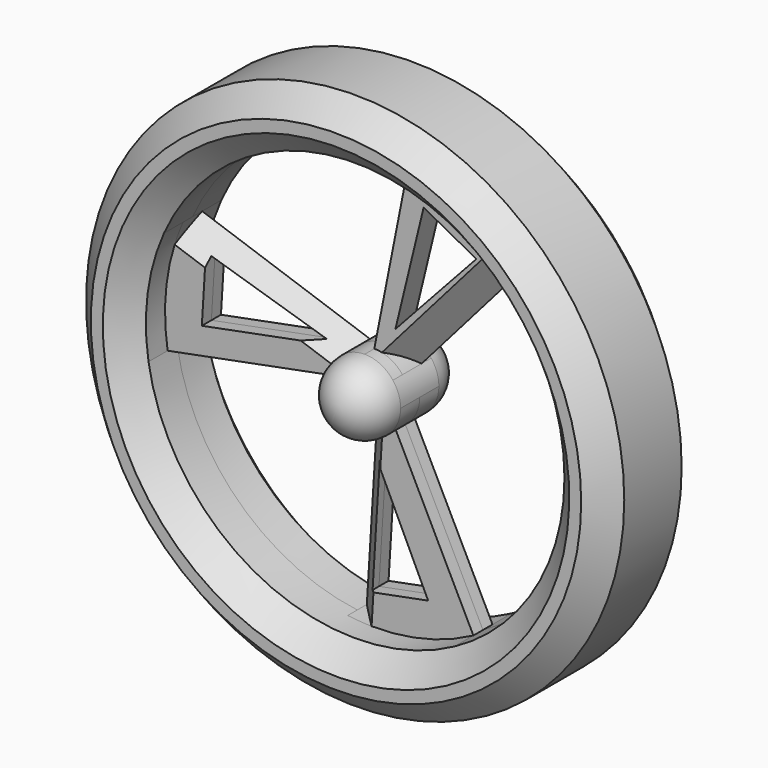
from build123d import *

# Parameters (mm, degrees)
F0_R          = 57.15
F1_DEPTH      = 12.7
F1_DEPTH_BACK = 12.7
F2_DEPTH      = 2.54
F2_DEPTH_BACK = 2.54
F4_T3_DEPTH   = 63.8207499086
F4_S4_R       = 7.62
F4_T5_DEPTH   = 35
F4_S6_R       = 44.45
F4_T7_DEPTH   = 35
F4_T10_DEPTH  = 63.0657347927
F4_S11_R      = 7.62
F4_T12_DEPTH  = 36
F4_S13_R      = 44.45
F4_T14_DEPTH  = 36
F4_T17_DEPTH  = 63.4473233417
F4_S18_R      = 7.62
F4_T19_DEPTH  = 34
F4_S20_R      = 44.45
F4_T21_DEPTH  = 34


# Not quite as in the source:
# - a fillet or chamfer that OpenCascade refuses, or shapes differently, is made with other operations: its cross-section is extruded or revolved along the edge and cut away or added


with BuildPart() as f1:
    # F0 (on Front) → F1 (new body, two sides)
    with BuildSketch(Plane.XZ) as f1_sk:
        Circle(F0_R)
        with BuildLine():
            ThreePointArc((30.2978338322, 32.5245102204), (40.7586875024, 17.7350470278), (44.45, 0))
            ThreePointArc((44.45, 0), (38.1514443262, -22.8094233996), (21.0407853398, -39.1546657793))
            ThreePointArc((21.0407853398, -39.1546657793), (8.0824234514, -43.7090028616), (-5.6476952972, -44.0897498046))
            ThreePointArc((-5.6476952972, -44.0897498046), (-30.9360762044, -31.9180464483), (-43.8918074796, -7.0222315665))
            ThreePointArc((-43.8918074796, -7.0222315665), (-44.0755738858, 5.7572811841), (-40.6153867658, 18.0608100003))
            ThreePointArc((-40.6153867658, 18.0608100003), (-21.1284803601, 39.1074138454), (7.15605679, 43.8701874992))
            ThreePointArc((7.15605679, 43.8701874992), (19.5673089339, 39.9114384743), (30.2978338322, 32.5245102204))
        make_face(mode=Mode.SUBTRACT)
    extrude(amount=F1_DEPTH)
    extrude(f1_sk.sketch, amount=-F1_DEPTH_BACK)



with BuildPart() as f1b:
    # F0 (on Front) → F1, piece 2 (new body, two sides)
    with BuildSketch(Plane.XZ) as f1_2_sk:
        with BuildLine():
            ThreePointArc((7.62, 0), (7.1992672661, 2.4969883522), (5.9835299656, 4.7182379285))
            ThreePointArc((5.9835299656, 4.7182379285), (3.3250133071, 6.8562880998), (0, 7.62))
            ThreePointArc((0, 7.62), (-2.66023415, 7.1405569998), (-4.9857096013, 5.7625601751))
            ThreePointArc((-4.9857096013, 5.7625601751), (-6.930205883, 3.168066669), (-7.62, 0))
            ThreePointArc((-7.62, 0), (-6.4667392377, -4.030593459), (-3.3560410415, -6.8411540348))
            ThreePointArc((-3.3560410415, -6.8411540348), (0.7135883563, -7.5865138013), (4.5728511754, -6.0953615256))
            ThreePointArc((4.5728511754, -6.0953615256), (6.815773102, -3.407291743), (7.62, 0))
        make_face()
    extrude(amount=F1_DEPTH)
    extrude(f1_2_sk.sketch, amount=-F1_DEPTH_BACK)


with BuildPart() as f1_1:
    add(f1.part)

    add(f1b.part)  # F2 merges F1b
    # F0 (on Front) → F2 (join, two sides)
    with BuildSketch(Plane.XZ) as f2_sk:
        with BuildLine():
            Line((5.9835299656, 4.7182379285), (30.2978338322, 32.5245102204))
            ThreePointArc((30.2978338322, 32.5245102204), (19.5673089339, 39.9114384743), (7.15605679, 43.8701874992))
            Line((7.15605679, 43.8701874992), (0, 7.62))
            ThreePointArc((0, 7.62), (3.3250133071, 6.8562880998), (5.9835299656, 4.7182379285))
        make_face()
        Polygon((21.6807832905, 31.4497899136), (4.4864523225, 12.7544701099), (10.4806591381, 37.4370446242), align=None, mode=Mode.SUBTRACT)
        with BuildLine():
            Line((-4.9857096013, 5.7625601751), (-40.6153867658, 18.0608100003))
            ThreePointArc((-40.6153867658, 18.0608100003), (-44.0755738858, 5.7572811841), (-43.8918074796, -7.0222315665))
            Line((-43.8918074796, -7.0222315665), (-7.62, 0))
            ThreePointArc((-7.62, 0), (-6.930205883, 3.168066669), (-4.9857096013, 5.7625601751))
        make_face()
        Polygon((-35.8506757944, 12.6760325764), (-11.6935795524, 4.8278034033), (-36.6305463748, 0), align=None, mode=Mode.SUBTRACT)
        with BuildLine():
            ThreePointArc((-5.6476952972, -44.0897498046), (8.0824234514, -43.7090028616), (21.0407853398, -39.1546657793))
            Line((21.0407853398, -39.1546657793), (4.5728511754, -6.0953615256))
            ThreePointArc((4.5728511754, -6.0953615256), (0.7135883563, -7.5865138013), (-3.3560410415, -6.8411540348))
            Line((-3.3560410415, -6.8411540348), (-5.6476952972, -44.0897498046))
        make_face()
        Polygon((-1.0400637192, -38.1721799109), (0.5196774415, -12.8201147581), (11.428419692, -35.7582782093), align=None, mode=Mode.SUBTRACT)
    extrude(amount=F2_DEPTH)
    extrude(f2_sk.sketch, amount=-F2_DEPTH_BACK)

    # F3: fillet of radius 7.62 on 2 edges, made by hand

    # F3_s1 → F3_t2 (revolve, cut)
    with BuildSketch(Plane(origin=(0, 0, 0), x_dir=(0, 1, 0), z_dir=(0.8977892434, 0, -0.4404253335))):
        with BuildLine():
            ThreePointArc((-5.08, -7.62), (-10.4681536726, -5.3881536726), (-12.7, 0))
            Line((-12.7, 0), (-12.7, -7.62))
            Line((-12.7, -7.62), (-5.08, -7.62))
        make_face()
    revolve(axis=Axis((0, -12.7, 0), (0, 1, 0)), mode=Mode.SUBTRACT)

    # F3_s3 → F3_t4 (revolve, cut)
    with BuildSketch(Plane(origin=(0, 0, 0), x_dir=(0, 1, 0), z_dir=(-0.8977892434, 0, 0.4404253335))):
        with BuildLine():
            ThreePointArc((5.08, 7.62), (10.4681536726, 5.3881536726), (12.7, 0))
            Line((12.7, 0), (12.7, 7.62))
            Line((12.7, 7.62), (5.08, 7.62))
        make_face()
    revolve(axis=Axis((0, 12.7, 0), (0, -1, 0)), mode=Mode.SUBTRACT)

    # F4: chamfer of 5.08 on 7 edges, made by hand


with BuildPart() as f4_tool1:
    # F4_s2 → F4_t3 (new body)
    with BuildSketch(Plane(origin=(6.116948919, 0, -2.1113793882), x_dir=(0, 1, 0), z_dir=(-0.9452735615, 0, 0.326278859))):
        Polygon((-2.54, 1.2595358599), (2.54, -3.8204641401), (-2.54, -3.8204641401), align=None)
    extrude(amount=F4_T3_DEPTH)

    # F4_s4 → F4_t5 (cut, symmetric)
    with BuildSketch(Plane.XZ):
        Circle(F4_S4_R)
    extrude(amount=F4_T5_DEPTH, both=True, mode=Mode.SUBTRACT)

    # F4_s6 → F4_t7 (intersect, symmetric)
    with BuildSketch(Plane.XZ):
        Circle(F4_S6_R)
    extrude(amount=F4_T7_DEPTH, both=True, mode=Mode.INTERSECT)


with BuildPart() as f4_tool8:
    # F4_s9 → F4_t10 (new body)
    with BuildSketch(Plane(origin=(-3.6688529254, 0, -4.1957657518), x_dir=(0, 1, 0), z_dir=(0.6582564125, 0, 0.7527937934))):
        Polygon((-2.54, 3.6814461509), (2.54, -1.3985538491), (-2.54, -1.3985538491), align=None)
    extrude(amount=F4_T10_DEPTH)

    # F4_s11 → F4_t12 (cut, symmetric)
    with BuildSketch(Plane.XZ):
        Circle(F4_S11_R)
    extrude(amount=F4_T12_DEPTH, both=True, mode=Mode.SUBTRACT)

    # F4_s13 → F4_t14 (intersect, symmetric)
    with BuildSketch(Plane.XZ):
        Circle(F4_S13_R)
    extrude(amount=F4_T14_DEPTH, both=True, mode=Mode.INTERSECT)


with BuildPart() as f4_tool15:
    # F4_s16 → F4_t17 (new body)
    with BuildSketch(Plane(origin=(0.3702740347, 0, 6.0184418339), x_dir=(0, 1, 0), z_dir=(-0.0614071323, 0, -0.9981128013))):
        Polygon((-2.54, 2.1503881258), (2.54, -2.9296118742), (-2.54, -2.9296118742), align=None)
    extrude(amount=F4_T17_DEPTH)

    # F4_s18 → F4_t19 (cut, symmetric)
    with BuildSketch(Plane.XZ):
        Circle(F4_S18_R)
    extrude(amount=F4_T19_DEPTH, both=True, mode=Mode.SUBTRACT)

    # F4_s20 → F4_t21 (intersect, symmetric)
    with BuildSketch(Plane.XZ):
        Circle(F4_S20_R)
    extrude(amount=F4_T21_DEPTH, both=True, mode=Mode.INTERSECT)


with BuildPart() as f4_tool22:
    # F4_s23 → F4_t24 (revolve)
    with BuildSketch(Plane(origin=(0, 0, 0), x_dir=(0, 1, 0), z_dir=(-0.8808698713, 0, -0.4733585003))):
        Polygon((-7.62, 44.45), (-12.7, 49.53), (-12.7, 44.45), align=None)
    revolve(axis=Axis((0, -12.7, 0), (0, -1, 0)))


with BuildPart() as f4_tool25:
    # F4_s26 → F4_t27 (revolve)
    with BuildSketch(Plane(origin=(0, 0, 0), x_dir=(0, 1, 0), z_dir=(0.8808698713, 0, 0.4733585003))):
        Polygon((7.62, -44.45), (12.7, -49.53), (12.7, -44.45), align=None)
    revolve(axis=Axis((0, 12.7, 0), (0, 1, 0)))


with BuildPart() as f4_tool28:
    # F4_s29 → F4_t30 (revolve)
    with BuildSketch(Plane.XY):
        Polygon((52.07, 12.7), (57.15, 7.62), (57.15, 12.7), align=None)
    revolve(axis=Axis((0, 12.7, 0), (0, -1, 0)))


with BuildPart() as f4_tool31:
    # F4_s32 → F4_t33 (revolve)
    with BuildSketch(Plane.XY):
        Polygon((52.07, -12.7), (57.15, -7.62), (57.15, -12.7), align=None)
    revolve(axis=Axis((0, -12.7, 0), (0, -1, 0)))


with BuildPart() as f1_2:
    add(f1_1.part)

    # F4_t34: cut F4_tool1, F4_tool8, F4_tool15, F4_tool22, F4_tool25, F4_tool28, F4_tool31
    add([f4_tool1.part, f4_tool8.part, f4_tool15.part, f4_tool22.part, f4_tool25.part, f4_tool28.part, f4_tool31.part], mode=Mode.SUBTRACT)


solid = f1_2.part
